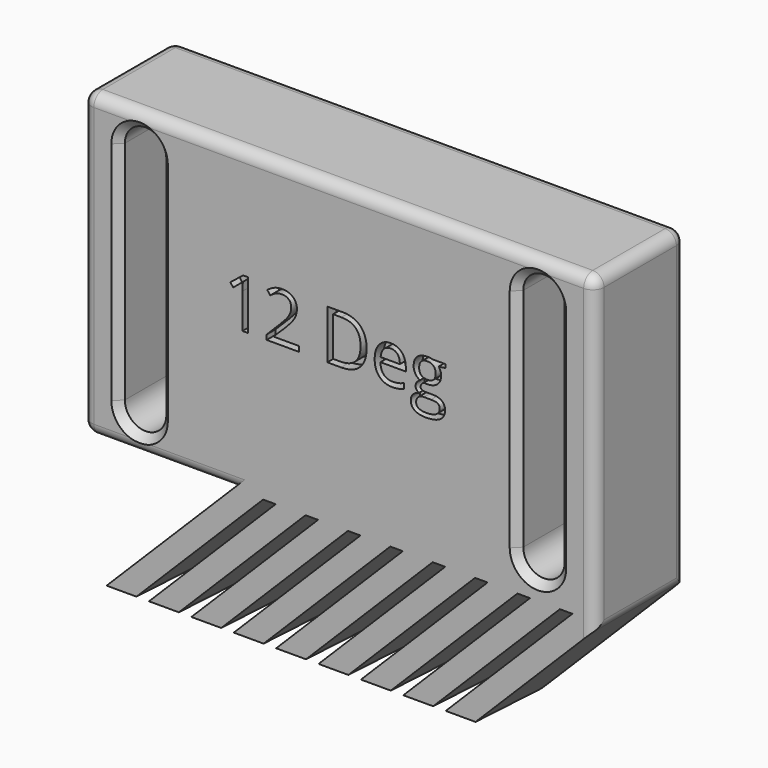
from build123d import *

# Parameters (mm, degrees)
F1_DEPTH     = 15
F2_SIZE      = 1
F3_T1_DEPTH  = 70.25
F3_T3_DEPTH  = 47.5
F3_T5_DEPTH  = 43.2097979746
F3_T7_DEPTH  = 12
F3_T9_DEPTH  = 18.1066017178
F3_S13_W     = 1.5
F3_S13_H     = 1.5
F3_T14_DEPTH = 1.5
F3_S19_W     = 1.5
F3_S19_H     = 1.5
F3_T20_DEPTH = 1.5
F3_T26_DEPTH = 27.5
F3_T31_DEPTH = 27.5
F5_DEPTH     = 35
F6_T1_DEPTH  = 12
F6_S5_W      = 1.5
F6_S5_H      = 1.5
F6_T6_DEPTH  = 1.5
F6_S11_W     = 1.5
F6_S11_H     = 1.5
F6_T12_DEPTH = 1.5
F6_S17_W     = 1.5
F6_S17_H     = 1.5
F6_T18_DEPTH = 1.5
F6_S23_W     = 1.5
F6_S23_H     = 1.5
F6_T24_DEPTH = 1.5
F7_TEXT_SIZE = 9.1402456441
F8_DEPTH     = 1.5


# Not quite as in the source:
# - a fillet or chamfer that OpenCascade refuses, or shapes differently, is made with other operations: its cross-section is extruded or revolved along the edge and cut away or added
# - Text() gives the source's letters only with a copy of the font that has no kerning and outlines rounded to 1/6400 em; it was checked with that copy


with BuildPart() as f1:
    # F0 (on Front) → F1 (new body)
    with BuildSketch(Plane.XZ):
        Polygon((34, -10.9597979746), (34, 30), (-34, 30), (-34, -10), (-14, -10), (-34, -30), (-30.0402020254, -30), (-10.0402020254, -10), (-8.375, -10), (-28.375, -30), (-24.4152020254, -30), (-4.4152020254, -10), (-2.75, -10), (-22.75, -30), (-18.7902020254, -30), (1.2097979746, -10), (2.875, -10), (-17.125, -30), (-13.1652020254, -30), (6.8347979746, -10), (8.5, -10), (-11.5, -30), (-7.5402020254, -30), (12.4597979746, -10), (14.125, -10), (-5.875, -30), (-1.9152020254, -30), (18.0847979746, -10), (19.75, -10), (-0.25, -30), (3.7097979746, -30), (23.7097979746, -10), (25.375, -10), (5.375, -30), (9.3347979746, -30), (29.3347979746, -10), (31, -10), (11, -30), (14.9597979746, -30), align=None)
        with BuildLine():
            Line((-29.1851401776, -5), (-29.1851401776, 25))
            ThreePointArc((-29.1851401776, 25), (-26.4351401776, 27.75), (-23.6851401776, 25))
            Line((-23.6851401776, 25), (-23.6851401776, -5))
            ThreePointArc((-23.6851401776, -5), (-26.4351401776, -7.75), (-29.1851401776, -5))
        make_face(mode=Mode.SUBTRACT)
        with BuildLine():
            Line((23.6851401776, -5), (23.6851401776, 25))
            ThreePointArc((23.6851401776, 25), (26.4351401776, 27.75), (29.1851401776, 25))
            Line((29.1851401776, 25), (29.1851401776, -5))
            ThreePointArc((29.1851401776, -5), (26.4351401776, -7.75), (23.6851401776, -5))
        make_face(mode=Mode.SUBTRACT)
    extrude(amount=F1_DEPTH)

    # F2
    f2_edges = [f1.edges().sort_by_distance(p)[0] for p in [
        (-29.18514, -15, 10),
        (-23.68514, 0, 10),
        (29.18514, 0, 10),
        (29.18514, -15, 10),
        (-29.18514, 0, 10),
        (-26.43514, 0, 27.75),
        (-26.43514, -15, 27.75),
        (-23.68514, -15, 10),
        (-26.43514, 0, -7.75),
        (-26.43514, -15, -7.75),
        (26.43514, 0, -7.75),
        (26.43514, -15, -7.75),
        (23.68514, 0, 10),
        (23.68514, -15, 10),
        (26.43514, 0, 27.75),
        (26.43514, -15, 27.75),
    ]]
    chamfer(f2_edges, length=F2_SIZE)

    # F3: fillet of radius 1.5 on 10 edges, made by hand

    # F3_s2 → F3_t1 (cut)
    with BuildSketch(Plane.YZ.offset(-37.75)):
        with BuildLine():
            ThreePointArc((-15, 28.5), (-14.5606601718, 29.5606601718), (-13.5, 30))
            Line((-13.5, 30), (-15, 30))
            Line((-15, 30), (-15, 28.5))
        make_face()
        with BuildLine():
            ThreePointArc((0, 28.5), (-0.4393398282, 29.5606601718), (-1.5, 30))
            Line((-1.5, 30), (0, 30))
            Line((0, 30), (0, 28.5))
        make_face()
    extrude(amount=F3_T1_DEPTH, mode=Mode.SUBTRACT)

    # F3_s4 → F3_t3 (cut)
    with BuildSketch(Plane.XY.offset(-13.75)):
        with BuildLine():
            ThreePointArc((-32.5, -15), (-33.5606601718, -14.5606601718), (-34, -13.5))
            Line((-34, -13.5), (-34, -15))
            Line((-34, -15), (-32.5, -15))
        make_face()
        with BuildLine():
            ThreePointArc((-32.5, 0), (-33.5606601718, -0.4393398282), (-34, -1.5))
            Line((-34, -1.5), (-34, 0))
            Line((-34, 0), (-32.5, 0))
        make_face()
    extrude(amount=F3_T3_DEPTH, mode=Mode.SUBTRACT)

    # F3_s6 → F3_t5 (cut)
    with BuildSketch(Plane.XY.offset(-14.7097979746)):
        with BuildLine():
            ThreePointArc((32.5, -15), (33.5606601718, -14.5606601718), (34, -13.5))
            Line((34, -13.5), (34, -15))
            Line((34, -15), (32.5, -15))
        make_face()
        with BuildLine():
            ThreePointArc((32.5, 0), (33.5606601718, -0.4393398282), (34, -1.5))
            Line((34, -1.5), (34, 0))
            Line((34, 0), (32.5, 0))
        make_face()
    extrude(amount=F3_T5_DEPTH, mode=Mode.SUBTRACT)

    # F3_s8 → F3_t7 (cut)
    with BuildSketch(Plane.XZ.offset(1.5)):
        with BuildLine():
            ThreePointArc((34, 28.5), (33.5606601718, 29.5606601718), (32.5, 30))
            Line((32.5, 30), (34, 30))
            Line((34, 30), (34, 28.5))
        make_face()
    extrude(amount=F3_T7_DEPTH, mode=Mode.SUBTRACT)

    # F3_s10 → F3_t9 (cut)
    with BuildSketch(Plane.XZ.offset(-1.5533008589)):
        with BuildLine():
            ThreePointArc((33.5606601718, -11.3991378029), (33.8858192988, -10.9125027796), (34, -10.3384776311))
            Line((34, -10.3384776311), (34, -10.9597979746))
            Line((34, -10.9597979746), (33.5606601718, -11.3991378029))
        make_face()
    extrude(amount=F3_T9_DEPTH, mode=Mode.SUBTRACT)


with BuildPart() as f3_tool12:
    # F3_s13 → F3_t14 (new body)
    with BuildSketch(Plane.XZ.offset(13.5)):
        with Locations((33.25, 29.25)):
            Rectangle(F3_S13_W, F3_S13_H)
    extrude(amount=F3_T14_DEPTH)

    # F3_s15 → F3_t16 (revolve, cut)
    with BuildSketch(Plane(origin=(32.5, -13.5, 28.5), x_dir=(-0.7071067812, 0, -0.7071067812), z_dir=(-0.7071067812, 0, 0.7071067812))):
        with BuildLine():
            ThreePointArc((0, -1.5), (1.5, 0), (0, 1.5))
            Line((0, 1.5), (0, -1.5))
        make_face()
    revolve(axis=Axis((32.5, -13.5, 28.5), (0, -1, 0)), mode=Mode.SUBTRACT)


with BuildPart() as f1_1:
    add(f1.part)

    # F3_t11: cut F3_tool12
    add(f3_tool12.part, mode=Mode.SUBTRACT)


with BuildPart() as f3_tool18:
    # F3_s19 → F3_t20 (new body)
    with BuildSketch(Plane.XZ.offset(1.5)):
        with Locations((33.25, 29.25)):
            Rectangle(F3_S19_W, F3_S19_H)
    extrude(amount=-F3_T20_DEPTH)

    # F3_s21 → F3_t22 (revolve, cut)
    with BuildSketch(Plane(origin=(32.5, -1.5, 28.5), x_dir=(-0.7071067812, 0, -0.7071067812), z_dir=(0.7071067812, 0, -0.7071067812))):
        with BuildLine():
            ThreePointArc((0, -1.5), (1.5, 0), (0, 1.5))
            Line((0, 1.5), (0, -1.5))
        make_face()
    revolve(axis=Axis((32.5, -1.5, 28.5), (0, 1, 0)), mode=Mode.SUBTRACT)


with BuildPart() as f1_2:
    add(f1_1.part)

    # F3_t17: cut F3_tool18
    add(f3_tool18.part, mode=Mode.SUBTRACT)


with BuildPart() as f3_tool24:
    # F3_s25 → F3_t26 (new body)
    with BuildSketch(Plane.YZ.offset(-37.75)):
        with BuildLine():
            ThreePointArc((-15, -8.5), (-14.5606601718, -9.5606601718), (-13.5, -10))
            Line((-13.5, -10), (-15, -10))
            Line((-15, -10), (-15, -8.5))
        make_face()
    extrude(amount=F3_T26_DEPTH)

    split(bisect_by=Plane(origin=(-2, 0, 2), x_dir=(0, 1, 0), z_dir=(-0.7071067812, 0, 0.7071067812)), keep=Keep.TOP)


with BuildPart() as f1_3:
    add(f1_2.part)

    # F3_t23: cut F3_tool24
    add(f3_tool24.part, mode=Mode.SUBTRACT)


with BuildPart() as f3_tool29:
    # F3_s30 → F3_t31 (new body)
    with BuildSketch(Plane.YZ.offset(-37.75)):
        with BuildLine():
            ThreePointArc((0, -8.5), (-0.4393398282, -9.5606601718), (-1.5, -10))
            Line((-1.5, -10), (0, -10))
            Line((0, -10), (0, -8.5))
        make_face()
    extrude(amount=F3_T31_DEPTH)

    split(bisect_by=Plane(origin=(-2, 0, 2), x_dir=(0, 1, 0), z_dir=(-0.7071067812, 0, 0.7071067812)), keep=Keep.TOP)


with BuildPart() as f1_4:
    add(f1_3.part)

    # F3_t28: cut F3_tool29
    add(f3_tool29.part, mode=Mode.SUBTRACT)

    # F4 (on Right) → F5 (cut, symmetric)
    with BuildSketch(Plane.YZ):
        Polygon((-15, -30), (0, -30), (-15, -26.8116515749), align=None)
    extrude(amount=F5_DEPTH, both=True, mode=Mode.SUBTRACT)

    # F6: fillet of radius 1.5 on 2 edges, made by hand

    # F6_s2 → F6_t1 (cut)
    with BuildSketch(Plane.XZ.offset(1.5)):
        with BuildLine():
            ThreePointArc((-34, 28.5), (-33.5606601718, 29.5606601718), (-32.5, 30))
            Line((-32.5, 30), (-34, 30))
            Line((-34, 30), (-34, 28.5))
        make_face()
        with BuildLine():
            ThreePointArc((-32.5, -10), (-33.5606601718, -9.5606601718), (-34, -8.5))
            Line((-34, -8.5), (-34, -10))
            Line((-34, -10), (-32.5, -10))
        make_face()
    extrude(amount=F6_T1_DEPTH, mode=Mode.SUBTRACT)


with BuildPart() as f6_tool4:
    # F6_s5 → F6_t6 (new body)
    with BuildSketch(Plane.XY.offset(-8.5)):
        with Locations((-33.25, -0.75)):
            Rectangle(F6_S5_W, F6_S5_H)
    extrude(amount=-F6_T6_DEPTH)

    # F6_s7 → F6_t8 (revolve, cut)
    with BuildSketch(Plane(origin=(-32.5, -1.5, -8.5), x_dir=(0.7071067812, -0.7071067812, 0), z_dir=(0.7071067812, 0.7071067812, 0))):
        with BuildLine():
            ThreePointArc((0, -1.5), (1.5, 0), (0, 1.5))
            Line((0, 1.5), (0, -1.5))
        make_face()
    revolve(axis=Axis((-32.5, -1.5, -8.5), (0, 0, -1)), mode=Mode.SUBTRACT)


with BuildPart() as f1_5:
    add(f1_4.part)

    # F6_t3: cut F6_tool4
    add(f6_tool4.part, mode=Mode.SUBTRACT)


with BuildPart() as f6_tool10:
    # F6_s11 → F6_t12 (new body)
    with BuildSketch(Plane.XY.offset(-8.5)):
        with Locations((-33.25, -14.25)):
            Rectangle(F6_S11_W, F6_S11_H)
    extrude(amount=-F6_T12_DEPTH)

    # F6_s13 → F6_t14 (revolve, cut)
    with BuildSketch(Plane(origin=(-32.5, -13.5, -8.5), x_dir=(0.7071067812, 0.7071067812, 0), z_dir=(-0.7071067812, 0.7071067812, 0))):
        with BuildLine():
            ThreePointArc((0, -1.5), (1.5, 0), (0, 1.5))
            Line((0, 1.5), (0, -1.5))
        make_face()
    revolve(axis=Axis((-32.5, -13.5, -8.5), (0, 0, -1)), mode=Mode.SUBTRACT)


with BuildPart() as f1_6:
    add(f1_5.part)

    # F6_t9: cut F6_tool10
    add(f6_tool10.part, mode=Mode.SUBTRACT)


with BuildPart() as f6_tool16:
    # F6_s17 → F6_t18 (new body)
    with BuildSketch(Plane.YZ.offset(-32.5)):
        with Locations((-0.75, 29.25)):
            Rectangle(F6_S17_W, F6_S17_H)
    extrude(amount=-F6_T18_DEPTH)

    # F6_s19 → F6_t20 (revolve, cut)
    with BuildSketch(Plane(origin=(-32.5, -1.5, 28.5), x_dir=(0, -0.7071067812, -0.7071067812), z_dir=(0, 0.7071067812, -0.7071067812))):
        with BuildLine():
            ThreePointArc((0, -1.5), (1.5, 0), (0, 1.5))
            Line((0, 1.5), (0, -1.5))
        make_face()
    revolve(axis=Axis((-32.5, -1.5, 28.5), (-1, 0, 0)), mode=Mode.SUBTRACT)


with BuildPart() as f1_7:
    add(f1_6.part)

    # F6_t15: cut F6_tool16
    add(f6_tool16.part, mode=Mode.SUBTRACT)


with BuildPart() as f6_tool22:
    # F6_s23 → F6_t24 (new body)
    with BuildSketch(Plane.YZ.offset(-32.5)):
        with Locations((-14.25, 29.25)):
            Rectangle(F6_S23_W, F6_S23_H)
    extrude(amount=-F6_T24_DEPTH)

    # F6_s25 → F6_t26 (revolve, cut)
    with BuildSketch(Plane(origin=(-32.5, -13.5, 28.5), x_dir=(0, 0.7071067812, -0.7071067812), z_dir=(0, 0.7071067812, 0.7071067812))):
        with BuildLine():
            ThreePointArc((0, -1.5), (1.5, 0), (0, 1.5))
            Line((0, 1.5), (0, -1.5))
        make_face()
    revolve(axis=Axis((-32.5, -13.5, 28.5), (-1, 0, 0)), mode=Mode.SUBTRACT)


with BuildPart() as f1_8:
    add(f1_7.part)

    # F6_t21: cut F6_tool22
    add(f6_tool22.part, mode=Mode.SUBTRACT)

    # F7 (on face) → F8 (cut)
    with BuildSketch(Plane.XZ.offset(15)):
        with Locations((-15.242151506, 8.8013301676)):
            Text('12 Deg', F7_TEXT_SIZE, font='Open Sans', text_align=(TextAlign.LEFT, TextAlign.BOTTOM))
    extrude(amount=-F8_DEPTH, mode=Mode.SUBTRACT)


solid = f1_8.part
